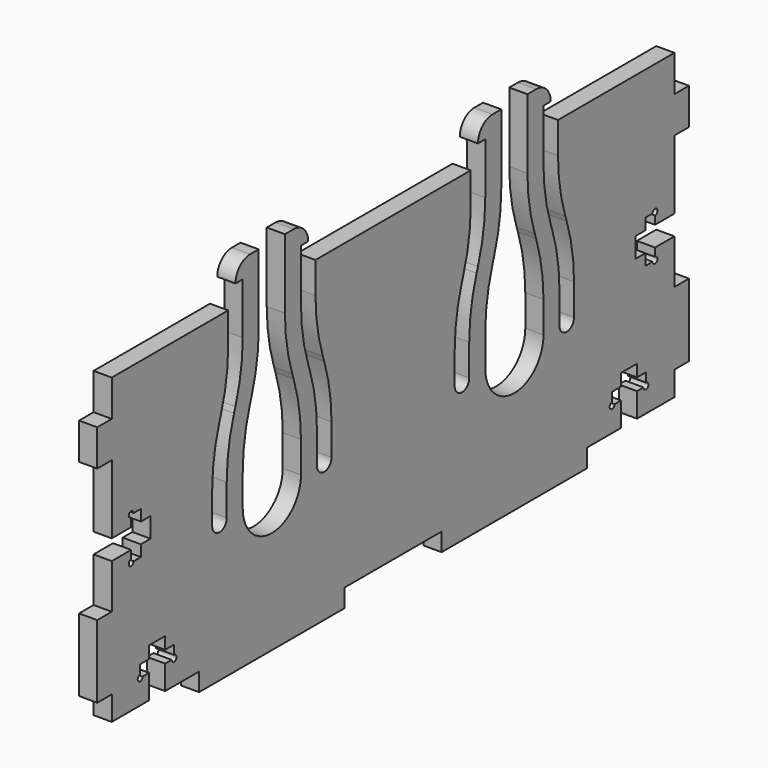
from build123d import *

# Parameters (mm, degrees)
F0_W     = 3
F0_H     = 6
F0_H_2   = 12
F0_W_2   = 30
F0_H_3   = 3
F1_DEPTH = 1.5


# Not quite as in the source:
# - a feature names something its author has since deleted; it is built from what else it names


with BuildPart() as f1:
    # F0 (on Right) → F1 (new body, symmetric)
    with BuildSketch(Plane.YZ):
        with BuildLine():
            Line((50.3, -25), (58, -25))
            Line((58, -25), (58, -21))
            Line((58, -21), (58, -9))
            Line((58, -9), (58, -1.65))
            Line((58, -1.65), (54, -1.65))
            Line((54, -1.65), (54, -3))
            ThreePointArc((54, -3), (54.3535533906, -3.1464466094), (54.5, -3.5))
            ThreePointArc((54.5, -3.5), (54, -4), (53.5, -3.5))
            Line((53.5, -3.5), (52, -3.5))
            Line((52, -3.5), (52, -1.65))
            Line((52, -1.65), (50, -1.65))
            Line((50, -1.65), (50, 1.65))
            Line((50, 1.65), (52, 1.65))
            Line((52, 1.65), (52, 3.5))
            Line((52, 3.5), (53.5, 3.5))
            ThreePointArc((53.5, 3.5), (54, 4), (54.5, 3.5))
            ThreePointArc((54.5, 3.5), (54.3535533906, 3.1464466094), (54, 3))
            Line((54, 3), (54, 1.65))
            Line((54, 1.65), (58, 1.65))
            Line((58, 1.65), (58, 13))
            Line((58, 13), (58, 19))
            Line((58, 19), (58, 25))
            Line((58, 25), (34, 25))
            Line((34, 25), (34, 19.8221099082))
            ThreePointArc((34, 19.8221099082), (34.3801942596, 15.0611112835), (35.5111405269, 10.4207862821))
            Line((35.5111405269, 10.4207862821), (35.7888594731, 9.5792137179))
            ThreePointArc((35.7888594731, 9.5792137179), (36.9198057404, 4.9388887165), (37.3, 0.1778900918))
            Line((37.3, 0.1778900918), (37.3, -5))
            ThreePointArc((37.3, -5), (35.8, -6.5), (34.3, -5))
            Line((34.3, -5), (34.3, 0.1778900918))
            ThreePointArc((34.3, 0.1778900918), (33.9198057404, 4.9388887165), (32.7888594731, 9.5792137179))
            Line((32.7888594731, 9.5792137179), (32.5111405269, 10.4207862821))
            ThreePointArc((32.5111405269, 10.4207862821), (31.3801942596, 15.0611112835), (31, 19.8221099082))
            Line((31, 19.8221099082), (31, 25))
            Line((31, 25), (27.7, 25))
            Line((27.7, 25), (27.7, 19.8221099082))
            ThreePointArc((27.7, 19.8221099082), (28.0801942596, 15.0611112835), (29.2111405269, 10.4207862821))
            Line((29.2111405269, 10.4207862821), (29.4888594731, 9.5792137179))
            ThreePointArc((29.4888594731, 9.5792137179), (30.6198057404, 4.9388887165), (31, 0.1778900918))
            Line((31, 0.1778900918), (31, -5))
            ThreePointArc((31, -5), (25, -11), (19, -5))
            Line((19, -5), (19, 0.1778900918))
            ThreePointArc((19, 0.1778900918), (19.3801942596, 4.9388887165), (20.5111405269, 9.5792137179))
            Line((20.5111405269, 9.5792137179), (20.7888594731, 10.4207862821))
            ThreePointArc((20.7888594731, 10.4207862821), (21.9198057404, 15.0611112835), (22.3, 19.8221099082))
            Line((22.3, 19.8221099082), (22.3, 25))
            Line((22.3, 25), (19, 25))
            Line((19, 25), (19, 19.8221099082))
            ThreePointArc((19, 19.8221099082), (18.6198057404, 15.0611112835), (17.4888594731, 10.4207862821))
            Line((17.4888594731, 10.4207862821), (17.2111405269, 9.5792137179))
            ThreePointArc((17.2111405269, 9.5792137179), (16.0801942596, 4.9388887165), (15.7, 0.1778900918))
            Line((15.7, 0.1778900918), (15.7, -5))
            ThreePointArc((15.7, -5), (14.2, -6.5), (12.7, -5))
            Line((12.7, -5), (12.7, 0.1778900918))
            ThreePointArc((12.7, 0.1778900918), (13.0801942596, 4.9388887165), (14.2111405269, 9.5792137179))
            Line((14.2111405269, 9.5792137179), (14.4888594731, 10.4207862821))
            ThreePointArc((14.4888594731, 10.4207862821), (15.6198057404, 15.0611112835), (16, 19.8221099082))
            Line((16, 19.8221099082), (16, 25))
            Line((16, 25), (-16, 25))
            Line((-16, 25), (-16, 19.8221099082))
            ThreePointArc((-16, 19.8221099082), (-15.6198057404, 15.0611112835), (-14.4888594731, 10.4207862821))
            Line((-14.4888594731, 10.4207862821), (-14.2111405269, 9.5792137179))
            ThreePointArc((-14.2111405269, 9.5792137179), (-13.0801942596, 4.9388887165), (-12.7, 0.1778900918))
            Line((-12.7, 0.1778900918), (-12.7, -5))
            ThreePointArc((-12.7, -5), (-14.2, -6.5), (-15.7, -5))
            Line((-15.7, -5), (-15.7, 0.1778900918))
            ThreePointArc((-15.7, 0.1778900918), (-16.0801942596, 4.9388887165), (-17.2111405269, 9.5792137179))
            Line((-17.2111405269, 9.5792137179), (-17.4888594731, 10.4207862821))
            ThreePointArc((-17.4888594731, 10.4207862821), (-18.6198057404, 15.0611112835), (-19, 19.8221099082))
            Line((-19, 19.8221099082), (-19, 25))
            Line((-19, 25), (-22.3, 25))
            Line((-22.3, 25), (-22.3, 19.8221099082))
            ThreePointArc((-22.3, 19.8221099082), (-21.9198057404, 15.0611112835), (-20.7888594731, 10.4207862821))
            Line((-20.7888594731, 10.4207862821), (-20.5111405269, 9.5792137179))
            ThreePointArc((-20.5111405269, 9.5792137179), (-19.3801942596, 4.9388887165), (-19, 0.1778900918))
            Line((-19, 0.1778900918), (-19, -5))
            ThreePointArc((-19, -5), (-25, -11), (-31, -5))
            Line((-31, -5), (-31, 0.1778900918))
            ThreePointArc((-31, 0.1778900918), (-30.6198057404, 4.9388887165), (-29.4888594731, 9.5792137179))
            Line((-29.4888594731, 9.5792137179), (-29.2111405269, 10.4207862821))
            ThreePointArc((-29.2111405269, 10.4207862821), (-28.0801942596, 15.0611112835), (-27.7, 19.8221099082))
            Line((-27.7, 19.8221099082), (-27.7, 25))
            Line((-27.7, 25), (-31, 25))
            Line((-31, 25), (-31, 19.8221099082))
            ThreePointArc((-31, 19.8221099082), (-31.3801942596, 15.0611112835), (-32.5111405269, 10.4207862821))
            Line((-32.5111405269, 10.4207862821), (-32.7888594731, 9.5792137179))
            ThreePointArc((-32.7888594731, 9.5792137179), (-33.9198057404, 4.9388887165), (-34.3, 0.1778900918))
            Line((-34.3, 0.1778900918), (-34.3, -5))
            ThreePointArc((-34.3, -5), (-35.8, -6.5), (-37.3, -5))
            Line((-37.3, -5), (-37.3, 0.1778900918))
            ThreePointArc((-37.3, 0.1778900918), (-36.9198057404, 4.9388887165), (-35.7888594731, 9.5792137179))
            Line((-35.7888594731, 9.5792137179), (-35.5111405269, 10.4207862821))
            ThreePointArc((-35.5111405269, 10.4207862821), (-34.3801942596, 15.0611112835), (-34, 19.8221099082))
            Line((-34, 19.8221099082), (-34, 25))
            Line((-34, 25), (-58, 25))
            Line((-58, 25), (-58, 19))
            Line((-58, 19), (-58, 13))
            Line((-58, 13), (-58, 1.65))
            Line((-58, 1.65), (-54, 1.65))
            Line((-54, 1.65), (-54, 3))
            ThreePointArc((-54, 3), (-54.3535533906, 3.8535533906), (-53.5, 3.5))
            Line((-53.5, 3.5), (-52, 3.5))
            Line((-52, 3.5), (-52, 1.65))
            Line((-52, 1.65), (-50, 1.65))
            Line((-50, 1.65), (-50, -1.65))
            Line((-50, -1.65), (-52, -1.65))
            Line((-52, -1.65), (-52, -3.5))
            Line((-52, -3.5), (-53.5, -3.5))
            ThreePointArc((-53.5, -3.5), (-54.3535533906, -3.8535533906), (-54, -3))
            Line((-54, -3), (-54, -1.65))
            Line((-54, -1.65), (-58, -1.65))
            Line((-58, -1.65), (-58, -9))
            Line((-58, -9), (-58, -21))
            Line((-58, -21), (-58, -25))
            Line((-58, -25), (-50.3, -25))
            Line((-50.3, -25), (-50.3, -21))
            Line((-50.3, -21), (-51.65, -21))
            ThreePointArc((-51.65, -21), (-52.5035533906, -21.3535533906), (-52.15, -20.5))
            Line((-52.15, -20.5), (-52.15, -19))
            Line((-52.15, -19), (-50.3, -19))
            Line((-50.3, -19), (-50.3, -17))
            Line((-50.3, -17), (-47, -17))
            Line((-47, -17), (-47, -19))
            Line((-47, -19), (-45.15, -19))
            Line((-45.15, -19), (-45.15, -20.5))
            ThreePointArc((-45.15, -20.5), (-44.7964466094, -20.6464466094), (-44.65, -21))
            ThreePointArc((-44.65, -21), (-45.15, -21.5), (-45.65, -21))
            Line((-45.65, -21), (-47, -21))
            Line((-47, -21), (-47, -25))
            Line((-47, -25), (-40, -25))
            Line((-40, -25), (-10, -25))
            Line((-10, -25), (10, -25))
            Line((10, -25), (40, -25))
            Line((40, -25), (47, -25))
            Line((47, -25), (47, -21))
            Line((47, -21), (45.65, -21))
            ThreePointArc((45.65, -21), (44.7964466094, -21.3535533906), (45.15, -20.5))
            Line((45.15, -20.5), (45.15, -19))
            Line((45.15, -19), (47, -19))
            Line((47, -19), (47, -17))
            Line((47, -17), (50.3, -17))
            Line((50.3, -17), (50.3, -19))
            Line((50.3, -19), (52.15, -19))
            Line((52.15, -19), (52.15, -20.5))
            ThreePointArc((52.15, -20.5), (52.5035533906, -20.6464466094), (52.65, -21))
            ThreePointArc((52.65, -21), (52.15, -21.5), (51.65, -21))
            Line((51.65, -21), (50.3, -21))
            Line((50.3, -21), (50.3, -25))
        make_face()
        with Locations((-59.5, 16)):
            Rectangle(F0_W, F0_H)
        with Locations((-59.5, -15)):
            Rectangle(F0_W, F0_H_2)
        with Locations((59.5, 16)):
            Rectangle(F0_W, F0_H)
        with Locations((59.5, -15)):
            Rectangle(F0_W, F0_H_2)
        with Locations((25, -26.5)):
            Rectangle(F0_W_2, F0_H_3)
        with Locations((-25, -26.5)):
            Rectangle(F0_W_2, F0_H_3)
        with BuildLine():
            Line((-31, 28.3), (-31, 25))
            Line((-31, 25), (-27.7, 25))
            Line((-27.7, 25), (-27.7, 31.3))
            Line((-27.7, 31.3), (-29.5, 31.3))
            ThreePointArc((-29.5, 31.3), (-31.6213203436, 30.4213203436), (-32.5, 28.3))
            Line((-32.5, 28.3), (-31, 28.3))
        make_face()
        with BuildLine():
            Line((-22.3, 25), (-19, 25))
            Line((-19, 25), (-19, 28.3))
            Line((-19, 28.3), (-17.5, 28.3))
            ThreePointArc((-17.5, 28.3), (-18.3786796564, 30.4213203436), (-20.5, 31.3))
            Line((-20.5, 31.3), (-22.3, 31.3))
            Line((-22.3, 31.3), (-22.3, 25))
        make_face()
        with BuildLine():
            Line((19, 25), (22.3, 25))
            Line((22.3, 25), (22.3, 31.3))
            Line((22.3, 31.3), (20.5, 31.3))
            ThreePointArc((20.5, 31.3), (18.3786796564, 30.4213203436), (17.5, 28.3))
            Line((17.5, 28.3), (19, 28.3))
            Line((19, 28.3), (19, 25))
        make_face()
        with BuildLine():
            Line((27.7, 25), (31, 25))
            Line((31, 25), (31, 28.3))
            Line((31, 28.3), (32.5, 28.3))
            ThreePointArc((32.5, 28.3), (31.6213203436, 30.4213203436), (29.5, 31.3))
            Line((29.5, 31.3), (27.7, 31.3))
            Line((27.7, 31.3), (27.7, 25))
        make_face()
    extrude(amount=F1_DEPTH, both=True)


solid = f1.part
